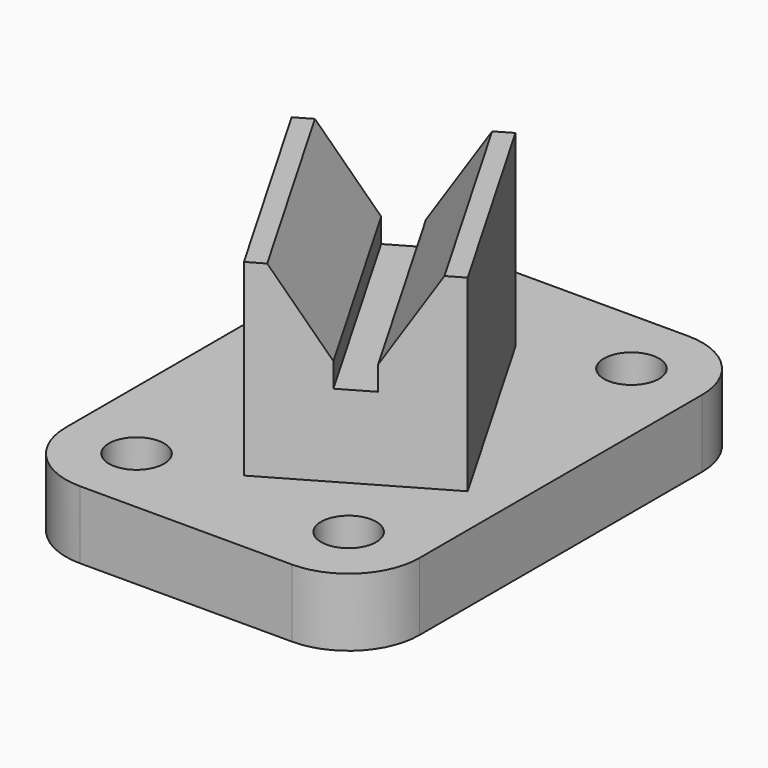
from build123d import *

# Parameters (mm, degrees)
F0_W     = 63.5
F0_H     = 88.9
F1_DEPTH = 12.192
F2_D     = 9.906
F6_DEPTH = 44.45
F7_R     = 12.7


# Not quite as in the source:
# - a pattern or mirror of a feature is missing from the dataset's text; its kind, count and spacing are read off the source's solid


with BuildPart() as f1:
    # F0 (on Top) → F1 (new body)
    with BuildSketch(Plane.XY):
        Rectangle(F0_W, F0_H)
    extrude(amount=-F1_DEPTH)

    # F2 (through all)
    with Locations(Plane.XY):
        with Locations((19.05, -31.75)):
            f2 = Hole(F2_D / 2)

    # F2_copies: F2 across plane
    add(f2.mirror(Plane(origin=(0, 0, 0), x_dir=(0.8574929257, 0.5144957554, 0), z_dir=(-0.5144957554, 0.8574929257, 0))), mode=Mode.SUBTRACT)

    # F2_copies1: F2 across plane
    add(f2.mirror(Plane(origin=(0, 0, 0), x_dir=(0, 0, -1), z_dir=(-1, 0, 0))), mode=Mode.SUBTRACT)

    # F2_copies2: F2 across plane
    add(f2.mirror(Plane.ZX), mode=Mode.SUBTRACT)

    # F5 (on line) → F6 (join, through all)
    with BuildSketch(Plane(origin=(11.1553204089, -19.3215817229, 0), x_dir=(0.8660254038, 0.5, 0), z_dir=(0.5, -0.8660254038, 0))):
        Polygon((-16.4748365541, 33.782), (-16.4748365541, 0), (15.2751634459, 0), (15.2751634459, 33.782), (11.9731634459, 33.782), (2.5751634459, 19.0759231813), (2.5751634459, 14.732), (-3.7748365541, 14.732), (-3.7748365541, 19.0759231813), (-13.1728365541, 33.782), align=None)
    extrude(amount=-F6_DEPTH)

    # F7
    f7_edges = [f1.edges().sort_by_distance(p)[0] for p in [
        (31.75, -44.45, -6.096),
        (31.75, 44.45, -6.096),
        (-31.75, 44.45, -6.096),
        (-31.75, -44.45, -6.096),
    ]]
    fillet(f7_edges, radius=F7_R)


solid = f1.part
